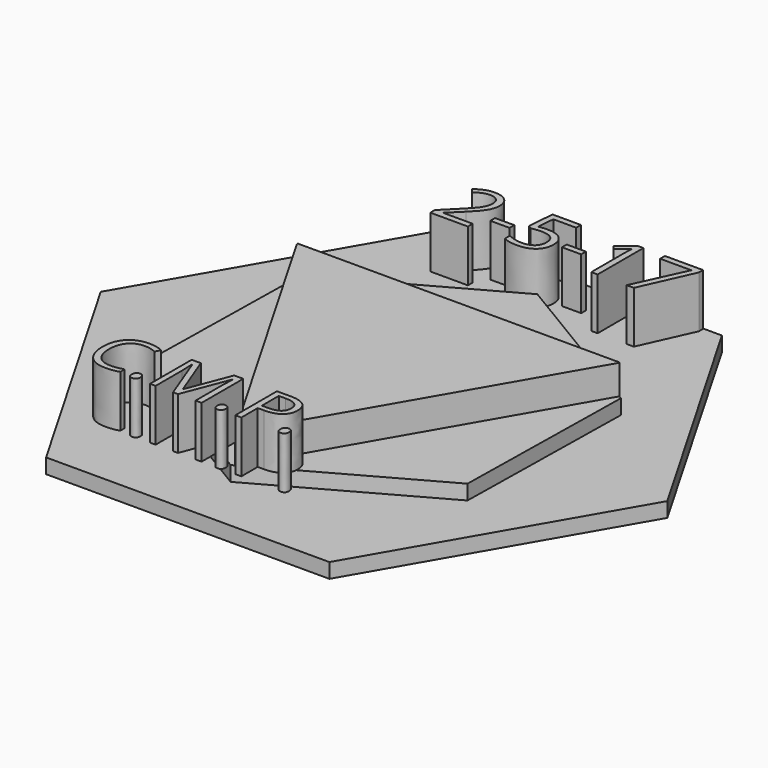
from build123d import *

# Parameters (mm, degrees)
F1_DEPTH      = 2
F3_DEPTH      = 2
F5_DEPTH      = 4
F8_TEXT_SIZE  = 9.8551261342
F9_DEPTH      = 7
F10_TEXT_SIZE = 10.8356286455
F11_DEPTH     = 7


# Not quite as in the source:
# - the program builds the solid bodies; features that only make, move or delete a surface that nothing else refers to are left out
# - Text() gives the source's letters only with a copy of the font that has no kerning and outlines rounded to 1/6400 em; it was checked with that copy


with BuildPart() as f1:
    # F0 (on Top) → F1 (new body)
    with BuildSketch(Plane.XY):
        Polygon((19.1414662904, 33.1539921463), (-19.1414662904, 33.1539921463), (-38.2829325807, 0), (-19.1414662904, -33.1539921463), (19.1414662904, -33.1539921463), (38.2829325807, 0), align=None)
    extrude(amount=F1_DEPTH)

    # F2 (on face) → F3 (join)
    with BuildSketch(Plane.XY.offset(2)):
        Polygon((0.4458033811, 25.3523395215), (-21.7328683805, 13.0622468139), (-22.1786717616, -12.2900927076), (-0.4458033811, -25.3523395215), (21.7328683805, -13.0622468139), (22.1786717616, 12.2900927076), align=None)
    extrude(amount=F3_DEPTH)

    # F4 (on face) → F5 (join)
    with BuildSketch(Plane.XY.offset(4)):
        Polygon((21.6614480918, 12.6009630039), (-21.7409797377, 12.6009630039), (-21.7434781194, 12.4588828283), (-0.0422642047, -25.128722258), (0.0820300277, -25.0598458322), (21.7832439424, 12.527759254), align=None)
    extrude(amount=F5_DEPTH)

    # F10 (on face) → F11 (join)
    with BuildSketch(Plane.XY.offset(2)):
        with Locations((-14.5583944395, 25.3523395215)):
            Text('2-5-17', F10_TEXT_SIZE, font='Open Sans', text_align=(TextAlign.LEFT, TextAlign.BOTTOM))
    extrude(amount=F11_DEPTH)


with BuildPart() as f9:
    # F8 (on face) → F9 (new body)
    with BuildSketch(Plane.XY.offset(8)):
        with Locations((-15.2924312279, -32.6646342874)):
            Text('C.M.P.', F8_TEXT_SIZE, font='Open Sans', text_align=(TextAlign.LEFT, TextAlign.BOTTOM))
    extrude(amount=F9_DEPTH)


solid = Compound([f1.part, f9.part])
